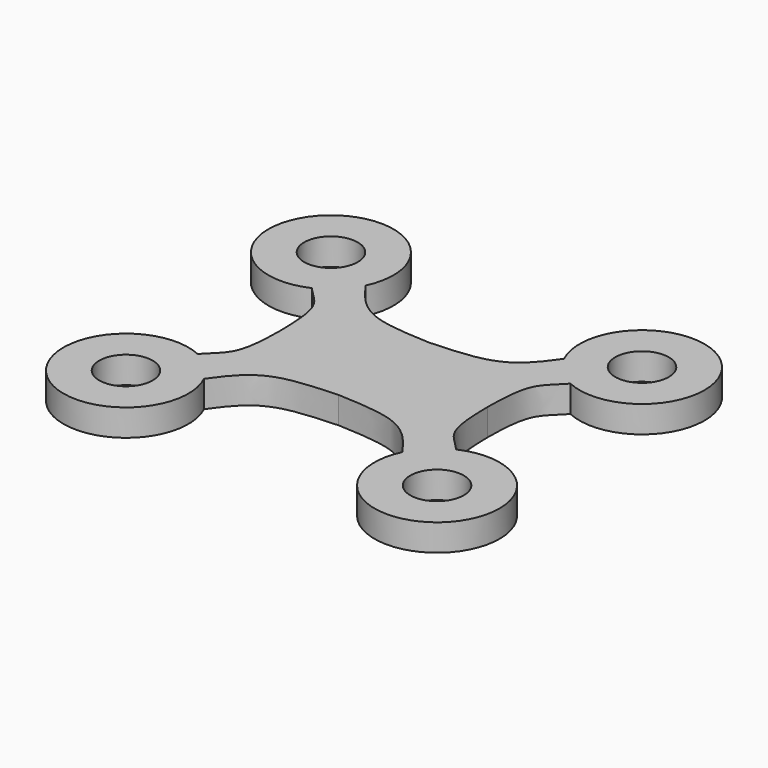
from build123d import *

# Parameters (mm, degrees)
F0_R     = 1.5
F1_DEPTH = 1.5


with BuildPart() as f1:
    # F0 (on Top) → F1 (new body)
    with BuildSketch(Plane.XY):
        with BuildLine():
            add(Edge.make_bspline(
                [(-5.5561550838, 5.6573497621), (-4.0955413133, 3.5522743128), (-3.2797986642, 3.3143495675), (0, 3.173440462)],
                knots=[0, 0, 0, 0, 6.0861042323, 6.0861042323, 6.0861042323, 6.0861042323], degree=3))
            ThreePointArc((-5.5561550838, 5.6573497621), (-11.1647533144, 9.6698318912), (-7.2436210565, 3.9969923231))
            add(Edge.make_bspline(
                [(-7.2436210565, 3.9969923231), (-6.2028751709, 2.9064782429), (-5.828993395, 2.9744568747), (-5.7950043119, 0)],
                knots=[0, 0, 0, 0, 4.2514042508, 4.2514042508, 4.2514042508, 4.2514042508], degree=3))
            add(Edge.make_bspline(
                [(-7.2436210565, -3.9969923231), (-6.2028751709, -2.9064782429), (-5.828993395, -2.9744568747), (-5.7950043119, 0)],
                knots=[0, 0, 0, 0, 4.2514042508, 4.2514042508, 4.2514042508, 4.2514042508], degree=3))
            ThreePointArc((-7.2436210565, -3.9969923231), (-11.1647533144, -9.6698318912), (-5.5561550838, -5.6573497621))
            add(Edge.make_bspline(
                [(-5.5561550838, -5.6573497621), (-4.0955413133, -3.5522743128), (-3.2797986642, -3.3143495675), (0, -3.173440462)],
                knots=[0, 0, 0, 0, 6.0861042323, 6.0861042323, 6.0861042323, 6.0861042323], degree=3))
            add(Edge.make_bspline(
                [(5.5561550838, -5.6573497621), (4.0955413133, -3.5522743128), (3.2797986642, -3.3143495675), (0, -3.173440462)],
                knots=[0, 0, 0, 0, 6.0861042323, 6.0861042323, 6.0861042323, 6.0861042323], degree=3))
            ThreePointArc((5.5561550838, -5.6573497621), (11.1647533144, -9.6698318912), (7.2436210565, -3.9969923231))
            add(Edge.make_bspline(
                [(7.2436210565, -3.9969923231), (6.2028751709, -2.9064782429), (5.828993395, -2.9744568747), (5.7950043119, 0)],
                knots=[0, 0, 0, 0, 4.2514042508, 4.2514042508, 4.2514042508, 4.2514042508], degree=3))
            add(Edge.make_bspline(
                [(7.2436210565, 3.9969923231), (6.2028751709, 2.9064782429), (5.828993395, 2.9744568747), (5.7950043119, 0)],
                knots=[0, 0, 0, 0, 4.2514042508, 4.2514042508, 4.2514042508, 4.2514042508], degree=3))
            ThreePointArc((7.2436210565, 3.9969923231), (11.1647533144, 9.6698318912), (5.5561550838, 5.6573497621))
            add(Edge.make_bspline(
                [(5.5561550838, 5.6573497621), (4.0955413133, 3.5522743128), (3.2797986642, 3.3143495675), (0, 3.173440462)],
                knots=[0, 0, 0, 0, 6.0861042323, 6.0861042323, 6.0861042323, 6.0861042323], degree=3))
        make_face()
        with Locations((-8.71, -7.175)):
            Circle(F0_R, mode=Mode.SUBTRACT)
        with Locations((8.71, -7.175)):
            Circle(F0_R, mode=Mode.SUBTRACT)
        with Locations((-8.71, 7.175)):
            Circle(F0_R, mode=Mode.SUBTRACT)
        with Locations((8.71, 7.175)):
            Circle(F0_R, mode=Mode.SUBTRACT)
    extrude(amount=F1_DEPTH)


solid = f1.part
